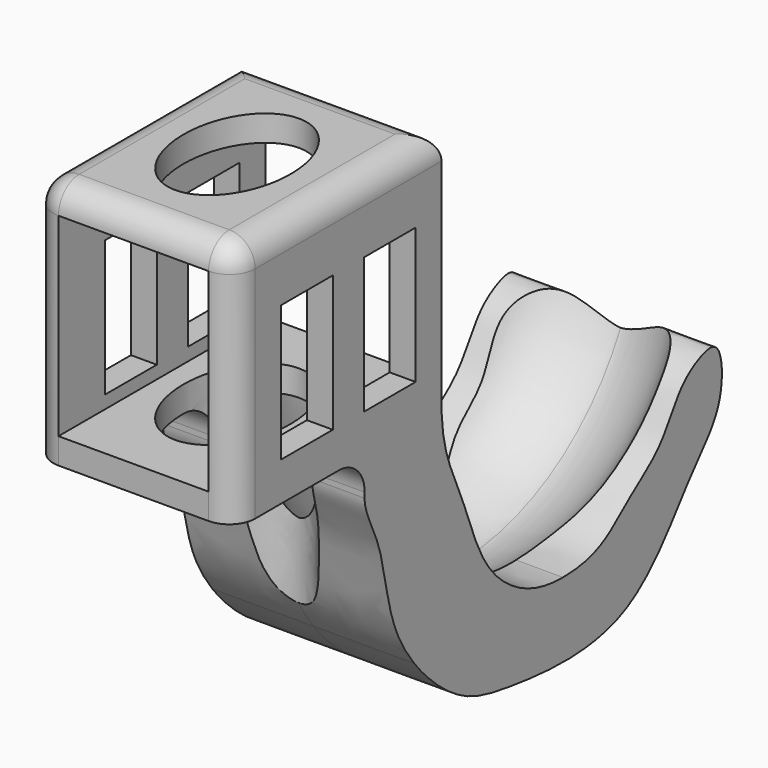
from build123d import *

# Parameters (mm, degrees)
F1_DEPTH      = 50.8
F3_DEPTH      = 19.812
F3_DEPTH_BACK = 19.812
F5_ANGLE      = 165
F6_R          = 5.07999
F8_DEPTH      = 39.6250001
F10_ANGLE     = 25
F12_DEPTH     = 117.4


# Not quite as in the source:
# - a fillet or chamfer is up to 0.001 mm smaller than in the source, because OpenCascade refuses the exact size


with BuildPart() as f1:
    # F0 (on Front) → F1 (new body)
    with BuildSketch(Plane.XZ):
        Polygon((-19.812, 0), (0, 0), (19.812, 0), (19.812, 48.26), (0, 48.26), (-19.812, 48.26), align=None)
        Polygon((0, 5.08), (-14.732, 5.08), (-14.732, 43.18), (0, 43.18), (14.732, 43.18), (14.732, 5.08), align=None, mode=Mode.SUBTRACT)
    extrude(amount=F1_DEPTH)

    # F2 (on Right) → F3 (join, two sides)
    with BuildSketch(Plane.YZ) as f3_sk:
        with BuildLine():
            add(Edge.make_bspline(
                [(0, 0), (0.3401417308, -7.8192657607), (4.9290795886, -15.0706707218), (9.7409360279, -31.9029741132), (20.2544577777, -39.8459897734), (26.6942867507, -40.8462825244), (29.8068448901, -40.8546999097)],
                knots=[0, 0, 0, 0, 0.0644956007, 0.1275724596, 0.1826651109, 0.2303740684, 0.2303740684, 0.2303740684, 0.2303740684], degree=3))
            Line((0, 0), (-25.2034073532, 0))
            ThreePointArc((-25.2034073532, 0), (-20.7132792926, -1.8598719395), (-18.8534073532, -6.35))
            Line((-18.8534073532, -6.35), (-18.8534073532, -7.3959506117))
            add(Edge.make_bspline(
                [(-6.7118525493, -40.8546999097), (-8.3306130442, -38.764736648), (-13.4514199568, -30.6561814823), (-13.8589057779, -17.3668520949), (-18.9147051903, -10.0806404002), (-18.8534073532, -7.3959506117)],
                knots=[0.8585533525, 0.8585533525, 0.8585533525, 0.8585533525, 0.8837704125, 0.9499094652, 1, 1, 1, 1], degree=3))
            Line((-6.7118525493, -40.8546999097), (29.8068448901, -40.8546999097))
        make_face()
        with BuildLine():
            add(Edge.make_bspline(
                [(29.8068448901, -40.8546999097), (32.9194033361, -40.8631172958), (39.4037031453, -39.9667697314), (46.239880616, -33.2358766515), (54.1722302834, -28.326417519), (58.0639376297, -19.7033933548), (63.2387936025, -16.2861190554), (68.7255121828, -15.0381122395), (69.5950266002, -27.6351598893), (59.8592325975, -36.3208962246), (46.7952486318, -57.8413431748), (24.6789394836, -55.5173462627), (16.8965887278, -54.4390156865)],
                knots=[0.2303740684, 0.2303740684, 0.2303740684, 0.2303740684, 0.2780830306, 0.3259594044, 0.3736629367, 0.4209482616, 0.4597588335, 0.4901193182, 0.5381324096, 0.5952001319, 0.6703761771, 0.7525068359, 0.7525068359, 0.7525068359, 0.7525068359], degree=3))
            Line((29.8068448901, -40.8546999097), (-6.7118525493, -40.8546999097))
            add(Edge.make_bspline(
                [(16.8965887278, -54.4390156865), (11.3411712787, -53.6692512944), (4.7626305756, -52.4013875119), (-3.6679654754, -44.7846278869), (-6.7118525493, -40.8546999097)],
                knots=[0.7525068359, 0.7525068359, 0.7525068359, 0.7525068359, 0.8111356628, 0.8585533525, 0.8585533525, 0.8585533525, 0.8585533525], degree=3))
        make_face()
    extrude(amount=F3_DEPTH)
    extrude(f3_sk.sketch, amount=-F3_DEPTH_BACK)

    # F4 (on Top) → F5 (revolve, cut)
    with BuildSketch(Plane.XY):
        with BuildLine():
            Line((16.9893931597, 3.3112922683), (0, 3.3112922683))
            Line((0, 3.3112922683), (-16.9893931597, 3.3112922683))
            add(Edge.make_bspline(
                [(-16.9893931597, 3.3112922683), (-17.3258762766, 3.2516035279), (-14.0834946023, 3.4169411442), (-15.1401046728, 0.9255223879), (-18.4108574597, -2.5434681452), (-13.2515389189, -12.0808145691), (-3.132803706, -15.2000690952), (0, -15.3263453394)],
                knots=[0, 0, 0, 0, 0.1241995958, 0.2375631302, 0.4160388116, 0.6834991086, 1, 1, 1, 1], degree=3))
            add(Edge.make_bspline(
                [(16.9893931597, 3.3112922683), (17.3258762766, 3.2516035279), (14.0834946023, 3.4169411442), (15.1401046728, 0.9255223879), (18.4108574597, -2.5434681452), (13.2515389189, -12.0808145691), (3.132803706, -15.2000690952), (0, -15.3263453394)],
                knots=[0, 0, 0, 0, 0.1241995958, 0.2375631302, 0.4160388116, 0.6834991086, 1, 1, 1, 1], degree=3))
        make_face()
    revolve(axis=Axis((3.1551243737, 29.0789715946, 0), (1, 0, 0)), revolution_arc=F5_ANGLE, mode=Mode.SUBTRACT)

    # F6 (radius 5.08 in the source; OpenCascade refuses exactly that, so slightly less here)
    f6_edges = [f1.edges().sort_by_distance(p)[0] for p in [
        (-19.812, -25.4, 48.26),
        (19.812, -25.4, 48.26),
        (-19.812, -50.8, 24.13),
        (19.812, -50.8, 24.13),
        (0, -50.8, 48.26),
        (0, 0, 48.26),
    ]]
    fillet(f6_edges, radius=F6_R)

    # F7 (on face) → F8 (cut, through all)
    with BuildSketch(Plane.YZ.offset(19.812)):
        Polygon((-26.67, 34.29), (-33.02, 34.29), (-39.37, 34.29), (-39.37, 7.62), (-33.02, 7.62), (-26.67, 7.62), align=None)
        Polygon((-12.7, 34.29), (-19.05, 34.29), (-19.05, 7.62), (-12.7, 7.62), (-6.35, 7.62), (-6.35, 34.29), align=None)
    extrude(amount=-F8_DEPTH, mode=Mode.SUBTRACT)

    # F9 (on face) → F10 (revolve)
    with BuildSketch(Plane.XY.offset(5.08)):
        with BuildLine():
            Line((-12.6549014822, -0.8907049121), (-16.1351338689, 0))
            add(Edge.make_bspline(
                [(-16.1351338689, 0), (-15.3500466409, -0.8907049121), (-13.3895511654, -2.6907462217), (-8.8969290781, -4.08677666), (0.0852984384, -5.5336293707), (7.0735466488, -4.5823116758), (10.548556368, -3.585144064), (11.5915354199, -3.2051558142)],
                knots=[0, 0, 0, 0, 0.135252337, 0.2876567768, 0.5015205789, 0.7051479963, 0.8049254223, 0.8049254223, 0.8049254223, 0.8049254223], degree=3))
            add(Edge.make_bspline(
                [(13.6379118559, -2.3219321916), (13.0485336228, -2.5743266081), (12.180913653, -2.9527613978), (11.5915354199, -3.2051558142)],
                knots=[0, 0, 0, 0, 2.2288428579, 2.2288428579, 2.2288428579, 2.2288428579], degree=3))
            add(Edge.make_bspline(
                [(13.6379118559, -2.3219321916), (14.7454411453, -1.7523842785), (15.6614363599, -1.0964802677), (15.6795078247, 0)],
                knots=[0.8752920454, 0.8752920454, 0.8752920454, 0.8752920454, 1, 1, 1, 1], degree=3))
            Line((15.6795078247, 0), (10.9098386019, -0.8972235955))
            add(Edge.make_bspline(
                [(-12.6549014822, -0.8907049121), (-11.9560259888, -1.2187900144), (-10.1642452035, -2.0599363812), (-3.409152494, -2.944084696), (-0.1182070998, -3.0059733591), (5.7662915833, -3.1941095747), (9.1887782032, -1.6657748472), (10.9098386019, -0.8972235955)],
                knots=[0, 0, 0, 0, 0.1515720858, 0.3886013368, 0.5631343004, 0.780314041, 1, 1, 1, 1], degree=3))
        make_face()
        with BuildLine():
            add(Edge.make_bspline(
                [(13.6379118559, -2.3219321916), (13.0485336228, -2.5743266081), (12.180913653, -2.9527613978), (11.5915354199, -3.2051558142)],
                knots=[0, 0, 0, 0, 2.2288428579, 2.2288428579, 2.2288428579, 2.2288428579], degree=3))
            add(Edge.make_bspline(
                [(11.5915354199, -3.2051558142), (12.3270816924, -2.9371744581), (13.0129870363, -2.6433003308), (13.6379118559, -2.3219321916)],
                knots=[0.8049254223, 0.8049254223, 0.8049254223, 0.8049254223, 0.8752920454, 0.8752920454, 0.8752920454, 0.8752920454], degree=3))
        make_face()
    revolve(axis=Axis((3.0634170398, 108.8161095977, 5.08), (1, 0, 0)), revolution_arc=F10_ANGLE)

    # F11 (on face) → F12 (cut)
    with BuildSketch(Plane.XY.offset(48.26)):
        with BuildLine():
            add(Edge.make_bspline(
                [(0, -10.2), (-18.2226913886, -10.2), (-9.1113456943, -33), (0, -55.8), (9.1113456943, -33), (18.2226913886, -10.2), (0, -10.2)],
                knots=[0, 0, 0, 2.0943951024, 2.0943951024, 4.1887902048, 4.1887902048, 6.2831853072, 6.2831853072, 6.2831853072], degree=2, weights=[1, 0.5, 1, 0.5, 1, 0.5, 1]))
        make_face()
    extrude(amount=-F12_DEPTH, mode=Mode.SUBTRACT)


solid = f1.part
